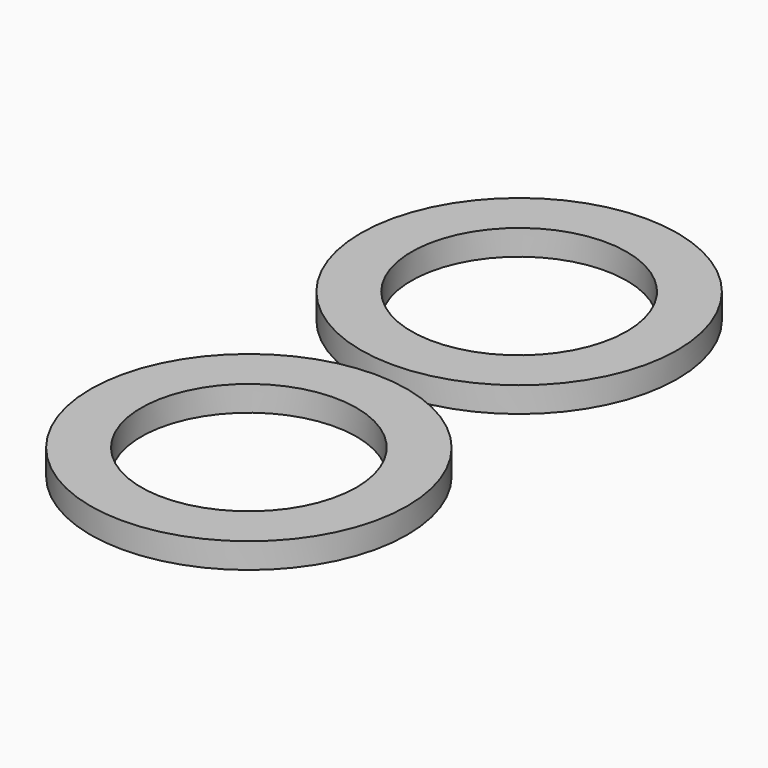
from build123d import *

# Parameters (mm, degrees)
F0_R     = 15
F0_R_2   = 10.2
F1_DEPTH = 2.4


# Not quite as in the source:
# - a feature names something its author has since deleted; it is built from what else it names


with BuildPart() as f1:
    # F0 (on Top) → F1 (new body)
    with BuildSketch(Plane.XY):
        with Locations((0, 32)):
            Circle(F0_R)
        with Locations((0, 32)):
            Circle(F0_R_2, mode=Mode.SUBTRACT)
    extrude(amount=F1_DEPTH)


with BuildPart() as f1b:
    # F0 (on Top) → F1, piece 2 (new body)
    with BuildSketch(Plane.XY):
        Circle(F0_R)
        Circle(F0_R_2, mode=Mode.SUBTRACT)
    extrude(amount=F1_DEPTH)


solid = Compound([f1.part, f1b.part])
